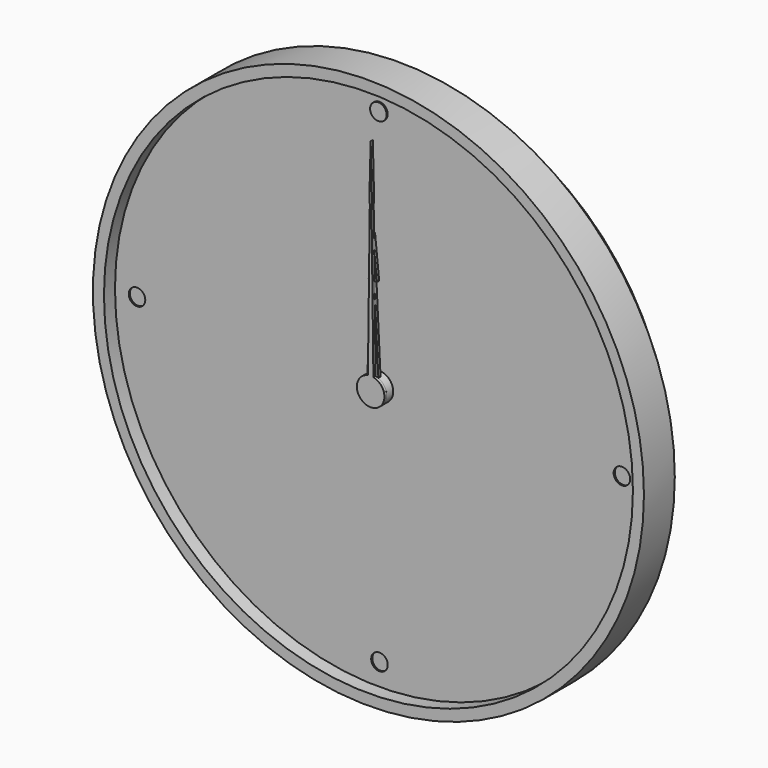
from build123d import *

# Parameters (mm, degrees)
F0_R      = 100
F1_DEPTH  = 24
F2_SIZE   = 10
F3_T      = -4
F4_R      = 5
F4_R_2    = 3
F5_DEPTH  = 2
F6_DEPTH  = 19
F7_DEPTH  = 8
F9_DEPTH  = 4
F11_DEPTH = 4
F12_R     = 5
F12_R_2   = 3
F13_DEPTH = 2
F14_R     = 3
F15_DEPTH = 4
F16_R     = 7.5
F17_DEPTH = 4
F18_R     = 3
F19_DEPTH = 2
F20_R     = 98
F20_R_2   = 5
F21_DEPTH = 1
F23_R     = 5
F23_R_2   = 3
F24_DEPTH = 2
F25_R     = 3
F26_DEPTH = 0.5
F27_DEPTH = 1
F28_R     = 5
F28_R_2   = 3
F29_DEPTH = 5
F30_R     = 3
F31_DEPTH = 1
F33_DEPTH = 1


with BuildPart() as f1:
    # F0 (on Front) → F1 (new body)
    with BuildSketch(Plane.XZ):
        Circle(F0_R)
    extrude(amount=F1_DEPTH)

    # F2
    f2_edges = [f1.edges().sort_by_distance(p)[0] for p in [
        (-100, 0, 0),
    ]]
    chamfer(f2_edges, length=F2_SIZE)

    # F3
    f3_openings = [f1.faces().sort_by_distance(p)[0] for p in [
        (0, -24, 0),
    ]]
    offset(amount=F3_T, openings=f3_openings)

    # F4 (on face) → F5 (join)
    with BuildSketch(Plane.XZ.offset(4)):
        Circle(F4_R)
        Circle(F4_R_2, mode=Mode.SUBTRACT)
        with Locations((40, 0)):
            Circle(F4_R)
        with Locations((40, 0)):
            Circle(F4_R_2, mode=Mode.SUBTRACT)
    extrude(amount=F5_DEPTH)


with BuildPart() as f6:
    # F6 (new): a face of the model
    f6_faces = [f1.part.faces().sort_by_distance(p)[0] for p in [
        (0, -4, 0),
    ]]
    extrude(f6_faces, amount=F6_DEPTH)

    # F8 (on face) → F9 (join)
    with BuildSketch(Plane.XZ.offset(6)):
        with BuildLine():
            ThreePointArc((9.2729637667, -1.3794085621), (9.3494561423, -0.6915886375), (9.375, 0))
            ThreePointArc((9.375, 0), (9.3494561423, 0.6915886375), (9.2729637667, 1.3794085621))
            ThreePointArc((9.2729637667, 1.3794085621), (8.9161548403, 2.8970343223), (8.3127812852, 4.3345463782))
            ThreePointArc((8.3127812852, 4.3345463782), (7.5845343223, 5.5104867402), (6.6911892658, 6.566476316))
            ThreePointArc((6.6911892658, 6.566476316), (5.5104867402, 7.5845343223), (4.1773988938, 8.3928519278))
            ThreePointArc((4.1773988938, 8.3928519278), (2.8970343223, 8.9161548403), (1.5536078905, 9.2453733036))
            ThreePointArc((1.5536078905, 9.2453733036), (0, 9.375), (-1.5536078905, 9.2453733036))
            ThreePointArc((-1.5536078905, 9.2453733036), (-2.8970343223, 8.9161548403), (-4.1773988938, 8.3928519278))
            ThreePointArc((-4.1773988938, 8.3928519278), (-5.5104867402, 7.5845343223), (-6.6911892658, 6.566476316))
            ThreePointArc((-6.6911892658, 6.566476316), (-7.5845343223, 5.5104867402), (-8.3127812852, 4.3345463782))
            ThreePointArc((-8.3127812852, 4.3345463782), (-8.9161548403, 2.8970343223), (-9.2729637667, 1.3794085621))
            ThreePointArc((-9.2729637667, 1.3794085621), (-9.375, 0), (-9.2729637667, -1.3794085621))
            ThreePointArc((-9.2729637667, -1.3794085621), (-8.9161548403, -2.8970343223), (-8.3127812852, -4.3345463782))
            ThreePointArc((-8.3127812852, -4.3345463782), (-7.5845343223, -5.5104867402), (-6.6911892658, -6.566476316))
            ThreePointArc((-6.6911892658, -6.566476316), (-5.5104867402, -7.5845343223), (-4.1773988938, -8.3928519278))
            ThreePointArc((-4.1773988938, -8.3928519278), (-2.8970343223, -8.9161548403), (-1.5536078905, -9.2453733036))
            ThreePointArc((-1.5536078905, -9.2453733036), (0, -9.375), (1.5536078905, -9.2453733036))
            ThreePointArc((1.5536078905, -9.2453733036), (2.8970343223, -8.9161548403), (4.1773988938, -8.3928519278))
            ThreePointArc((4.1773988938, -8.3928519278), (5.5104867402, -7.5845343223), (6.6911892658, -6.566476316))
            ThreePointArc((6.6911892658, -6.566476316), (7.5845343223, -5.5104867402), (8.3127812852, -4.3345463782))
            ThreePointArc((8.3127812852, -4.3345463782), (8.9161548403, -2.8970343223), (9.2729637667, -1.3794085621))
        make_face()
        with BuildLine():
            ThreePointArc((8.3127812852, 4.3345463782), (8.9161548403, 2.8970343223), (9.2729637667, 1.3794085621))
            Line((9.2729637667, 1.3794085621), (11.1823199426, 2.3946312492))
            Line((11.1823199426, 2.3946312492), (10.8182678729, 3.515068311))
            Line((10.8182678729, 3.515068311), (10.4542158031, 4.6355053728))
            Line((10.4542158031, 4.6355053728), (8.3127812852, 4.3345463782))
        make_face()
        with BuildLine():
            Line((11.1823199426, -2.3946312492), (9.2729637667, -1.3794085621))
            ThreePointArc((9.2729637667, -1.3794085621), (8.9161548403, -2.8970343223), (8.3127812852, -4.3345463782))
            Line((8.3127812852, -4.3345463782), (10.4542158031, -4.6355053728))
            Line((10.4542158031, -4.6355053728), (10.8182678729, -3.515068311))
            Line((10.8182678729, -3.515068311), (11.1823199426, -2.3946312492))
        make_face()
        with BuildLine():
            ThreePointArc((4.1773988938, 8.3928519278), (5.5104867402, 7.5845343223), (6.6911892658, 6.566476316))
            Line((6.6911892658, 6.566476316), (7.6391579371, 8.5101001246))
            Line((7.6391579371, 8.5101001246), (6.6860572448, 9.202568311))
            Line((6.6860572448, 9.202568311), (5.7329565525, 9.8950364974))
            Line((5.7329565525, 9.8950364974), (4.1773988938, 8.3928519278))
        make_face()
        with BuildLine():
            Line((7.6391579371, -8.5101001246), (6.6911892658, -6.566476316))
            ThreePointArc((6.6911892658, -6.566476316), (5.5104867402, -7.5845343223), (4.1773988938, -8.3928519278))
            Line((4.1773988938, -8.3928519278), (5.7329565525, -9.8950364974))
            Line((5.7329565525, -9.8950364974), (6.6860572448, -9.202568311))
            Line((6.6860572448, -9.202568311), (7.6391579371, -8.5101001246))
        make_face()
        with BuildLine():
            ThreePointArc((-1.5536078905, 9.2453733036), (0, 9.375), (1.5536078905, 9.2453733036))
            Line((1.5536078905, 9.2453733036), (1.1780972451, 11.375))
            Line((1.1780972451, 11.375), (0, 11.375))
            Line((0, 11.375), (-1.1780972451, 11.375))
            Line((-1.1780972451, 11.375), (-1.5536078905, 9.2453733036))
        make_face()
        with BuildLine():
            Line((1.1780972451, -11.375), (1.5536078905, -9.2453733036))
            ThreePointArc((1.5536078905, -9.2453733036), (0, -9.375), (-1.5536078905, -9.2453733036))
            Line((-1.5536078905, -9.2453733036), (-1.1780972451, -11.375))
            Line((-1.1780972451, -11.375), (0, -11.375))
            Line((0, -11.375), (1.1780972451, -11.375))
        make_face()
        with BuildLine():
            ThreePointArc((-6.6911892658, 6.566476316), (-5.5104867402, 7.5845343223), (-4.1773988938, 8.3928519278))
            Line((-4.1773988938, 8.3928519278), (-5.7329565525, 9.8950364974))
            Line((-5.7329565525, 9.8950364974), (-6.6860572448, 9.202568311))
            Line((-6.6860572448, 9.202568311), (-7.6391579371, 8.5101001246))
            Line((-7.6391579371, 8.5101001246), (-6.6911892658, 6.566476316))
        make_face()
        with BuildLine():
            Line((-5.7329565525, -9.8950364974), (-4.1773988938, -8.3928519278))
            ThreePointArc((-4.1773988938, -8.3928519278), (-5.5104867402, -7.5845343223), (-6.6911892658, -6.566476316))
            Line((-6.6911892658, -6.566476316), (-7.6391579371, -8.5101001246))
            Line((-7.6391579371, -8.5101001246), (-6.6860572448, -9.202568311))
            Line((-6.6860572448, -9.202568311), (-5.7329565525, -9.8950364974))
        make_face()
        with BuildLine():
            ThreePointArc((-9.2729637667, 1.3794085621), (-8.9161548403, 2.8970343223), (-8.3127812852, 4.3345463782))
            Line((-8.3127812852, 4.3345463782), (-10.4542158031, 4.6355053728))
            Line((-10.4542158031, 4.6355053728), (-10.8182678729, 3.515068311))
            Line((-10.8182678729, 3.515068311), (-11.1823199426, 2.3946312492))
            Line((-11.1823199426, 2.3946312492), (-9.2729637667, 1.3794085621))
        make_face()
        with BuildLine():
            Line((-10.4542158031, -4.6355053728), (-8.3127812852, -4.3345463782))
            ThreePointArc((-8.3127812852, -4.3345463782), (-8.9161548403, -2.8970343223), (-9.2729637667, -1.3794085621))
            Line((-9.2729637667, -1.3794085621), (-11.1823199426, -2.3946312492))
            Line((-11.1823199426, -2.3946312492), (-10.8182678729, -3.515068311))
            Line((-10.8182678729, -3.515068311), (-10.4542158031, -4.6355053728))
        make_face()
    extrude(amount=F9_DEPTH)

    # F32 (on face) → F33 (join)
    with BuildSketch(Plane.XZ.offset(23)):
        with BuildLine():
            ThreePointArc((-1, 4.8989794856), (-3.1622776602, -3.8729833462), (5, 0))
            ThreePointArc((5, 0), (3.8729833462, 3.1622776602), (1, 4.8989794856))
            ThreePointArc((1, 4.8989794856), (0, 5), (-1, 4.8989794856))
        make_face()
        with BuildLine():
            ThreePointArc((-1, 4.8989794856), (0, 5), (1, 4.8989794856))
            Line((1, 4.8989794856), (0.3, 60.0062509769))
            Line((0.3, 60.0062509769), (0.5, 60.0062509769))
            Line((0.5, 60.0062509769), (0, 80))
            Line((0, 80), (-0.5, 60.0062509769))
            Line((-0.5, 60.0062509769), (-0.3, 60.0062509769))
            Line((-0.3, 60.0062509769), (-1, 4.8989794856))
        make_face()
    extrude(amount=-F33_DEPTH)


with BuildPart() as f7:
    # F7 (new): a face of the model
    f7_faces = [f1.part.faces().sort_by_distance(p)[0] for p in [
        (40, -4, 0),
    ]]
    extrude(f7_faces, amount=F7_DEPTH)

    # F10 (on face) → F11 (join)
    with BuildSketch(Plane.XZ.offset(6)):
        with BuildLine():
            ThreePointArc((68.0829066802, -1.5381733945), (68.1144747006, -0.7693746225), (68.125, 0))
            ThreePointArc((68.125, 0), (68.1144747006, 0.7693746225), (68.0829066802, 1.5381733945))
            ThreePointArc((68.0829066802, 1.5381733945), (67.9709283072, 2.9398630294), (67.7890320221, 4.3342039956))
            ThreePointArc((67.7890320221, 4.3342039956), (67.5104012706, 5.8475163042), (67.1494235596, 7.3433252263))
            ThreePointArc((67.1494235596, 7.3433252263), (66.7484645208, 8.6911029668), (66.280643318, 10.0171558733))
            ThreePointArc((66.280643318, 10.0171558733), (65.6934659962, 11.4394680865), (65.0293803521, 12.8275385085))
            ThreePointArc((65.0293803521, 12.8275385085), (64.3569644814, 14.0625), (63.6236643925, 15.2623099717))
            ThreePointArc((63.6236643925, 15.2623099717), (62.7536029668, 16.5314602207), (61.815433119, 17.7511268046))
            ThreePointArc((61.815433119, 17.7511268046), (60.9009482166, 18.8192983038), (59.934217974, 19.8404278876))
            ThreePointArc((59.934217974, 19.8404278876), (58.8192983038, 20.9009482166), (57.6480467764, 21.8989056799))
            ThreePointArc((57.6480467764, 21.8989056799), (56.5314602207, 22.7536029668), (55.3735505752, 23.5514238999))
            ThreePointArc((55.3735505752, 23.5514238999), (54.0625, 24.3569644814), (52.709356105, 25.0895972944))
            ThreePointArc((52.709356105, 25.0895972944), (51.4394680865, 25.6934659962), (50.1409852457, 26.2331096755))
            ThreePointArc((50.1409852457, 26.2331096755), (48.6911029668, 26.7484645208), (47.2152055856, 27.1837531139))
            ThreePointArc((47.2152055856, 27.1837531139), (45.8475163042, 27.5104012706), (44.4652101991, 27.7682826779))
            ThreePointArc((44.4652101991, 27.7682826779), (42.9398630294, 27.9709283072), (41.4057159597, 28.0898484802))
            ThreePointArc((41.4057159597, 28.0898484802), (40, 28.125), (38.5942840403, 28.0898484802))
            ThreePointArc((38.5942840403, 28.0898484802), (37.0601369706, 27.9709283072), (35.5347898009, 27.7682826779))
            ThreePointArc((35.5347898009, 27.7682826779), (34.1524836958, 27.5104012706), (32.7847944144, 27.1837531139))
            ThreePointArc((32.7847944144, 27.1837531139), (31.3088970332, 26.7484645208), (29.8590147543, 26.2331096755))
            ThreePointArc((29.8590147543, 26.2331096755), (28.5605319135, 25.6934659962), (27.290643895, 25.0895972944))
            ThreePointArc((27.290643895, 25.0895972944), (25.9375, 24.3569644814), (24.6264494248, 23.5514238999))
            ThreePointArc((24.6264494248, 23.5514238999), (23.4685397793, 22.7536029668), (22.3519532236, 21.8989056799))
            ThreePointArc((22.3519532236, 21.8989056799), (21.1807016962, 20.9009482166), (20.065782026, 19.8404278876))
            ThreePointArc((20.065782026, 19.8404278876), (19.0990517834, 18.8192983038), (18.184566881, 17.7511268046))
            ThreePointArc((18.184566881, 17.7511268046), (17.2463970332, 16.5314602207), (16.3763356075, 15.2623099717))
            ThreePointArc((16.3763356075, 15.2623099717), (15.6430355186, 14.0625), (14.9706196479, 12.8275385085))
            ThreePointArc((14.9706196479, 12.8275385085), (14.3065340038, 11.4394680865), (13.719356682, 10.0171558733))
            ThreePointArc((13.719356682, 10.0171558733), (13.2515354792, 8.6911029668), (12.8505764404, 7.3433252263))
            ThreePointArc((12.8505764404, 7.3433252263), (12.4895987294, 5.8475163042), (12.2109679779, 4.3342039956))
            ThreePointArc((12.2109679779, 4.3342039956), (12.0290716928, 2.9398630294), (11.9170933198, 1.5381733945))
            ThreePointArc((11.9170933198, 1.5381733945), (11.875, 0), (11.9170933198, -1.5381733945))
            ThreePointArc((11.9170933198, -1.5381733945), (12.0290716928, -2.9398630294), (12.2109679779, -4.3342039956))
            ThreePointArc((12.2109679779, -4.3342039956), (12.4895987294, -5.8475163042), (12.8505764404, -7.3433252263))
            ThreePointArc((12.8505764404, -7.3433252263), (13.2515354792, -8.6911029668), (13.719356682, -10.0171558733))
            ThreePointArc((13.719356682, -10.0171558733), (14.3065340038, -11.4394680865), (14.9706196479, -12.8275385085))
            ThreePointArc((14.9706196479, -12.8275385085), (15.6430355186, -14.0625), (16.3763356075, -15.2623099717))
            ThreePointArc((16.3763356075, -15.2623099717), (17.2463970332, -16.5314602207), (18.184566881, -17.7511268046))
            ThreePointArc((18.184566881, -17.7511268046), (19.0990517834, -18.8192983038), (20.065782026, -19.8404278876))
            ThreePointArc((20.065782026, -19.8404278876), (21.1807016962, -20.9009482166), (22.3519532236, -21.8989056799))
            ThreePointArc((22.3519532236, -21.8989056799), (23.4685397793, -22.7536029668), (24.6264494248, -23.5514238999))
            ThreePointArc((24.6264494248, -23.5514238999), (25.9375, -24.3569644814), (27.290643895, -25.0895972944))
            ThreePointArc((27.290643895, -25.0895972944), (28.5605319135, -25.6934659962), (29.8590147543, -26.2331096755))
            ThreePointArc((29.8590147543, -26.2331096755), (31.3088970332, -26.7484645208), (32.7847944144, -27.1837531139))
            ThreePointArc((32.7847944144, -27.1837531139), (34.1524836958, -27.5104012706), (35.5347898009, -27.7682826779))
            ThreePointArc((35.5347898009, -27.7682826779), (37.0601369706, -27.9709283072), (38.5942840403, -28.0898484802))
            ThreePointArc((38.5942840403, -28.0898484802), (40, -28.125), (41.4057159597, -28.0898484802))
            ThreePointArc((41.4057159597, -28.0898484802), (42.9398630294, -27.9709283072), (44.4652101991, -27.7682826779))
            ThreePointArc((44.4652101991, -27.7682826779), (45.8475163042, -27.5104012706), (47.2152055856, -27.1837531139))
            ThreePointArc((47.2152055856, -27.1837531139), (48.6911029668, -26.7484645208), (50.1409852457, -26.2331096755))
            ThreePointArc((50.1409852457, -26.2331096755), (51.4394680865, -25.6934659962), (52.709356105, -25.0895972944))
            ThreePointArc((52.709356105, -25.0895972944), (54.0625, -24.3569644814), (55.3735505752, -23.5514238999))
            ThreePointArc((55.3735505752, -23.5514238999), (56.5314602207, -22.7536029668), (57.6480467764, -21.8989056799))
            ThreePointArc((57.6480467764, -21.8989056799), (58.8192983038, -20.9009482166), (59.934217974, -19.8404278876))
            ThreePointArc((59.934217974, -19.8404278876), (60.9009482166, -18.8192983038), (61.815433119, -17.7511268046))
            ThreePointArc((61.815433119, -17.7511268046), (62.7536029668, -16.5314602207), (63.6236643925, -15.2623099717))
            ThreePointArc((63.6236643925, -15.2623099717), (64.3569644814, -14.0625), (65.0293803521, -12.8275385085))
            ThreePointArc((65.0293803521, -12.8275385085), (65.6934659962, -11.4394680865), (66.280643318, -10.0171558733))
            ThreePointArc((66.280643318, -10.0171558733), (66.7484645208, -8.6911029668), (67.1494235596, -7.3433252263))
            ThreePointArc((67.1494235596, -7.3433252263), (67.5104012706, -5.8475163042), (67.7890320221, -4.3342039956))
            ThreePointArc((67.7890320221, -4.3342039956), (67.9709283072, -2.9398630294), (68.0829066802, -1.5381733945))
        make_face()
        with BuildLine():
            ThreePointArc((68.0829066802, 1.5381733945), (68.1144747006, 0.7693746225), (68.125, 0))
            ThreePointArc((68.125, 0), (68.1144747006, -0.7693746225), (68.0829066802, -1.5381733945))
            Line((68.0829066802, -1.5381733945), (70.125, -1.1780972451))
            Line((70.125, -1.1780972451), (70.125, 0))
            Line((70.125, 0), (70.125, 1.1780972451))
            Line((70.125, 1.1780972451), (68.0829066802, 1.5381733945))
        make_face()
        with BuildLine():
            ThreePointArc((67.1494235596, 7.3433252263), (67.5104012706, 5.8475163042), (67.7890320221, 4.3342039956))
            Line((67.7890320221, 4.3342039956), (69.7116366623, 5.1109866922))
            Line((69.7116366623, 5.1109866922), (69.4666964721, 6.2633396859))
            Line((69.4666964721, 6.2633396859), (69.2217562819, 7.4156926796))
            Line((69.2217562819, 7.4156926796), (67.1494235596, 7.3433252263))
        make_face()
        with BuildLine():
            Line((69.7116366623, -5.1109866922), (67.7890320221, -4.3342039956))
            ThreePointArc((67.7890320221, -4.3342039956), (67.5104012706, -5.8475163042), (67.1494235596, -7.3433252263))
            Line((67.1494235596, -7.3433252263), (69.2217562819, -7.4156926796))
            Line((69.2217562819, -7.4156926796), (69.4666964721, -6.2633396859))
            Line((69.4666964721, -6.2633396859), (69.7116366623, -5.1109866922))
        make_face()
        with BuildLine():
            ThreePointArc((65.0293803521, 12.8275385085), (65.6934659962, 11.4394680865), (66.280643318, 10.0171558733))
            Line((66.280643318, 10.0171558733), (67.9997322302, 11.1766959857))
            Line((67.9997322302, 11.1766959857), (67.5205569115, 12.2529413727))
            Line((67.5205569115, 12.2529413727), (67.0413815928, 13.3291867596))
            Line((67.0413815928, 13.3291867596), (65.0293803521, 12.8275385085))
        make_face()
        with BuildLine():
            Line((67.9997322302, -11.1766959857), (66.280643318, -10.0171558733))
            ThreePointArc((66.280643318, -10.0171558733), (65.6934659962, -11.4394680865), (65.0293803521, -12.8275385085))
            Line((65.0293803521, -12.8275385085), (67.0413815928, -13.3291867596))
            Line((67.0413815928, -13.3291867596), (67.5205569115, -12.2529413727))
            Line((67.5205569115, -12.2529413727), (67.9997322302, -11.1766959857))
        make_face()
        with BuildLine():
            ThreePointArc((61.815433119, 17.7511268046), (62.7536029668, 16.5314602207), (63.6236643925, 15.2623099717))
            Line((63.6236643925, 15.2623099717), (65.064105142, 16.753930033))
            Line((65.064105142, 16.753930033), (64.3716369555, 17.7070307253))
            Line((64.3716369555, 17.7070307253), (63.6791687691, 18.6601314176))
            Line((63.6791687691, 18.6601314176), (61.815433119, 17.7511268046))
        make_face()
        with BuildLine():
            Line((65.064105142, -16.753930033), (63.6236643925, -15.2623099717))
            ThreePointArc((63.6236643925, -15.2623099717), (62.7536029668, -16.5314602207), (61.815433119, -17.7511268046))
            Line((61.815433119, -17.7511268046), (63.6791687691, -18.6601314176))
            Line((63.6791687691, -18.6601314176), (64.3716369555, -17.7070307253))
            Line((64.3716369555, -17.7070307253), (65.064105142, -16.753930033))
        make_face()
        with BuildLine():
            ThreePointArc((57.6480467764, 21.8989056799), (58.8192983038, 20.9009482166), (59.934217974, 19.8404278876))
            Line((59.934217974, 19.8404278876), (61.0330563882, 21.5989369435))
            Line((61.0330563882, 21.5989369435), (60.1575595166, 22.3872378675))
            Line((60.1575595166, 22.3872378675), (59.282062645, 23.1755387915))
            Line((59.282062645, 23.1755387915), (57.6480467764, 21.8989056799))
        make_face()
        with BuildLine():
            Line((61.0330563882, -21.5989369435), (59.934217974, -19.8404278876))
            ThreePointArc((59.934217974, -19.8404278876), (58.8192983038, -20.9009482166), (57.6480467764, -21.8989056799))
            Line((57.6480467764, -21.8989056799), (59.282062645, -23.1755387915))
            Line((59.282062645, -23.1755387915), (60.1575595166, -22.3872378675))
            Line((60.1575595166, -22.3872378675), (61.0330563882, -21.5989369435))
        make_face()
        with BuildLine():
            ThreePointArc((52.709356105, 25.0895972944), (54.0625, 24.3569644814), (55.3735505752, 23.5514238999))
            Line((55.3735505752, 23.5514238999), (56.0827621424, 25.4999666665))
            Line((56.0827621424, 25.4999666665), (55.0625, 26.089015289))
            Line((55.0625, 26.089015289), (54.0422378576, 26.6780639116))
            Line((54.0422378576, 26.6780639116), (52.709356105, 25.0895972944))
        make_face()
        with BuildLine():
            Line((56.0827621424, -25.4999666665), (55.3735505752, -23.5514238999))
            ThreePointArc((55.3735505752, -23.5514238999), (54.0625, -24.3569644814), (52.709356105, -25.0895972944))
            Line((52.709356105, -25.0895972944), (54.0422378576, -26.6780639116))
            Line((54.0422378576, -26.6780639116), (55.0625, -26.089015289))
            Line((55.0625, -26.089015289), (56.0827621424, -25.4999666665))
        make_face()
        with BuildLine():
            ThreePointArc((47.2152055856, 27.1837531139), (48.6911029668, 26.7484645208), (50.1409852457, 26.2331096755))
            Line((50.1409852457, 26.2331096755), (50.4295740173, 28.2865254836))
            Line((50.4295740173, 28.2865254836), (49.3091369555, 28.6505775534))
            Line((49.3091369555, 28.6505775534), (48.1886998938, 29.0146296232))
            Line((48.1886998938, 29.0146296232), (47.2152055856, 27.1837531139))
        make_face()
        with BuildLine():
            Line((50.4295740173, -28.2865254836), (50.1409852457, -26.2331096755))
            ThreePointArc((50.1409852457, -26.2331096755), (48.6911029668, -26.7484645208), (47.2152055856, -27.1837531139))
            Line((47.2152055856, -27.1837531139), (48.1886998938, -29.0146296232))
            Line((48.1886998938, -29.0146296232), (49.3091369555, -28.6505775534))
            Line((49.3091369555, -28.6505775534), (50.4295740173, -28.2865254836))
        make_face()
        with BuildLine():
            ThreePointArc((41.4057159597, 28.0898484802), (42.9398630294, 27.9709283072), (44.4652101991, 27.7682826779))
            Line((44.4652101991, 27.7682826779), (44.3205634611, 29.8368274034))
            Line((44.3205634611, 29.8368274034), (43.1489199559, 29.959972098))
            Line((43.1489199559, 29.959972098), (41.9772764508, 30.0831167926))
            Line((41.9772764508, 30.0831167926), (41.4057159597, 28.0898484802))
        make_face()
        with BuildLine():
            Line((44.3205634611, -29.8368274034), (44.4652101991, -27.7682826779))
            ThreePointArc((44.4652101991, -27.7682826779), (42.9398630294, -27.9709283072), (41.4057159597, -28.0898484802))
            Line((41.4057159597, -28.0898484802), (41.9772764508, -30.0831167926))
            Line((41.9772764508, -30.0831167926), (43.1489199559, -29.959972098))
            Line((43.1489199559, -29.959972098), (44.3205634611, -29.8368274034))
        make_face()
        with BuildLine():
            ThreePointArc((35.5347898009, 27.7682826779), (37.0601369706, 27.9709283072), (38.5942840403, 28.0898484802))
            Line((38.5942840403, 28.0898484802), (38.0227235492, 30.0831167926))
            Line((38.0227235492, 30.0831167926), (36.8510800441, 29.959972098))
            Line((36.8510800441, 29.959972098), (35.6794365389, 29.8368274034))
            Line((35.6794365389, 29.8368274034), (35.5347898009, 27.7682826779))
        make_face()
        with BuildLine():
            Line((38.0227235492, -30.0831167926), (38.5942840403, -28.0898484802))
            ThreePointArc((38.5942840403, -28.0898484802), (37.0601369706, -27.9709283072), (35.5347898009, -27.7682826779))
            Line((35.5347898009, -27.7682826779), (35.6794365389, -29.8368274034))
            Line((35.6794365389, -29.8368274034), (36.8510800441, -29.959972098))
            Line((36.8510800441, -29.959972098), (38.0227235492, -30.0831167926))
        make_face()
        with BuildLine():
            ThreePointArc((29.8590147543, 26.2331096755), (31.3088970332, 26.7484645208), (32.7847944144, 27.1837531139))
            Line((32.7847944144, 27.1837531139), (31.8113001062, 29.0146296232))
            Line((31.8113001062, 29.0146296232), (30.6908630445, 28.6505775534))
            Line((30.6908630445, 28.6505775534), (29.5704259827, 28.2865254836))
            Line((29.5704259827, 28.2865254836), (29.8590147543, 26.2331096755))
        make_face()
        with BuildLine():
            Line((31.8113001062, -29.0146296232), (32.7847944144, -27.1837531139))
            ThreePointArc((32.7847944144, -27.1837531139), (31.3088970332, -26.7484645208), (29.8590147543, -26.2331096755))
            Line((29.8590147543, -26.2331096755), (29.5704259827, -28.2865254836))
            Line((29.5704259827, -28.2865254836), (30.6908630445, -28.6505775534))
            Line((30.6908630445, -28.6505775534), (31.8113001062, -29.0146296232))
        make_face()
        with BuildLine():
            ThreePointArc((24.6264494248, 23.5514238999), (25.9375, 24.3569644814), (27.290643895, 25.0895972944))
            Line((27.290643895, 25.0895972944), (25.9577621424, 26.6780639116))
            Line((25.9577621424, 26.6780639116), (24.9375, 26.089015289))
            Line((24.9375, 26.089015289), (23.9172378576, 25.4999666665))
            Line((23.9172378576, 25.4999666665), (24.6264494248, 23.5514238999))
        make_face()
        with BuildLine():
            Line((25.9577621424, -26.6780639116), (27.290643895, -25.0895972944))
            ThreePointArc((27.290643895, -25.0895972944), (25.9375, -24.3569644814), (24.6264494248, -23.5514238999))
            Line((24.6264494248, -23.5514238999), (23.9172378576, -25.4999666665))
            Line((23.9172378576, -25.4999666665), (24.9375, -26.089015289))
            Line((24.9375, -26.089015289), (25.9577621424, -26.6780639116))
        make_face()
        with BuildLine():
            ThreePointArc((20.065782026, 19.8404278876), (21.1807016962, 20.9009482166), (22.3519532236, 21.8989056799))
            Line((22.3519532236, 21.8989056799), (20.717937355, 23.1755387915))
            Line((20.717937355, 23.1755387915), (19.8424404834, 22.3872378675))
            Line((19.8424404834, 22.3872378675), (18.9669436118, 21.5989369435))
            Line((18.9669436118, 21.5989369435), (20.065782026, 19.8404278876))
        make_face()
        with BuildLine():
            Line((20.717937355, -23.1755387915), (22.3519532236, -21.8989056799))
            ThreePointArc((22.3519532236, -21.8989056799), (21.1807016962, -20.9009482166), (20.065782026, -19.8404278876))
            Line((20.065782026, -19.8404278876), (18.9669436118, -21.5989369435))
            Line((18.9669436118, -21.5989369435), (19.8424404834, -22.3872378675))
            Line((19.8424404834, -22.3872378675), (20.717937355, -23.1755387915))
        make_face()
        with BuildLine():
            ThreePointArc((16.3763356075, 15.2623099717), (17.2463970332, 16.5314602207), (18.184566881, 17.7511268046))
            Line((18.184566881, 17.7511268046), (16.3208312309, 18.6601314176))
            Line((16.3208312309, 18.6601314176), (15.6283630445, 17.7070307253))
            Line((15.6283630445, 17.7070307253), (14.935894858, 16.753930033))
            Line((14.935894858, 16.753930033), (16.3763356075, 15.2623099717))
        make_face()
        with BuildLine():
            Line((16.3208312309, -18.6601314176), (18.184566881, -17.7511268046))
            ThreePointArc((18.184566881, -17.7511268046), (17.2463970332, -16.5314602207), (16.3763356075, -15.2623099717))
            Line((16.3763356075, -15.2623099717), (14.935894858, -16.753930033))
            Line((14.935894858, -16.753930033), (15.6283630445, -17.7070307253))
            Line((15.6283630445, -17.7070307253), (16.3208312309, -18.6601314176))
        make_face()
        with BuildLine():
            ThreePointArc((13.719356682, 10.0171558733), (14.3065340038, 11.4394680865), (14.9706196479, 12.8275385085))
            Line((14.9706196479, 12.8275385085), (12.9586184072, 13.3291867596))
            Line((12.9586184072, 13.3291867596), (12.4794430885, 12.2529413727))
            Line((12.4794430885, 12.2529413727), (12.0002677698, 11.1766959857))
            Line((12.0002677698, 11.1766959857), (13.719356682, 10.0171558733))
        make_face()
        with BuildLine():
            Line((12.9586184072, -13.3291867596), (14.9706196479, -12.8275385085))
            ThreePointArc((14.9706196479, -12.8275385085), (14.3065340038, -11.4394680865), (13.719356682, -10.0171558733))
            Line((13.719356682, -10.0171558733), (12.0002677698, -11.1766959857))
            Line((12.0002677698, -11.1766959857), (12.4794430885, -12.2529413727))
            Line((12.4794430885, -12.2529413727), (12.9586184072, -13.3291867596))
        make_face()
        with BuildLine():
            ThreePointArc((12.2109679779, 4.3342039956), (12.4895987294, 5.8475163042), (12.8505764404, 7.3433252263))
            Line((12.8505764404, 7.3433252263), (10.7782437181, 7.4156926796))
            Line((10.7782437181, 7.4156926796), (10.5333035279, 6.2633396859))
            Line((10.5333035279, 6.2633396859), (10.2883633377, 5.1109866922))
            Line((10.2883633377, 5.1109866922), (12.2109679779, 4.3342039956))
        make_face()
        with BuildLine():
            Line((10.7782437181, -7.4156926796), (12.8505764404, -7.3433252263))
            ThreePointArc((12.8505764404, -7.3433252263), (12.4895987294, -5.8475163042), (12.2109679779, -4.3342039956))
            Line((12.2109679779, -4.3342039956), (10.2883633377, -5.1109866922))
            Line((10.2883633377, -5.1109866922), (10.5333035279, -6.2633396859))
            Line((10.5333035279, -6.2633396859), (10.7782437181, -7.4156926796))
        make_face()
        with BuildLine():
            ThreePointArc((11.9170933198, -1.5381733945), (11.875, 0), (11.9170933198, 1.5381733945))
            Line((11.9170933198, 1.5381733945), (9.875, 1.1780972451))
            Line((9.875, 1.1780972451), (9.875, 0))
            Line((9.875, 0), (9.875, -1.1780972451))
            Line((9.875, -1.1780972451), (11.9170933198, -1.5381733945))
        make_face()
    extrude(amount=F11_DEPTH)

    # F16 (on face) → F17 (join)
    with BuildSketch(Plane.XZ.offset(12)):
        with Locations((40, 0)):
            Circle(F16_R)
    extrude(amount=F17_DEPTH)

    # F18 (on face) → F19 (join)
    with BuildSketch(Plane.XZ.offset(16)):
        with Locations((40, 0)):
            Circle(F18_R)
    extrude(amount=F19_DEPTH)


with BuildPart() as f13:
    # F12 (on face) → F13 (new body)
    with BuildSketch(Plane.XZ.offset(10)):
        Circle(F12_R)
        Circle(F12_R_2, mode=Mode.SUBTRACT)
    extrude(amount=F13_DEPTH)

    # F14 (on face) → F15 (join)
    with BuildSketch(Plane.XZ.offset(12)):
        with BuildLine():
            ThreePointArc((29.9718156995, -1.3001014101), (29.9929530972, -0.6502034357), (30, 0))
            ThreePointArc((30, 0), (29.9929530972, 0.6502034357), (29.9718156995, 1.3001014101))
            ThreePointArc((29.9718156995, 1.3001014101), (29.907520012, 2.3537728718), (29.8061935814, 3.4045299509))
            ThreePointArc((29.8061935814, 3.4045299509), (29.6306502179, 4.6930339512), (29.3994322443, 5.9727199596))
            ThreePointArc((29.3994322443, 5.9727199596), (29.1710976119, 7.0033609157), (28.9066440563, 8.0253304855))
            ThreePointArc((28.9066440563, 8.0253304855), (28.5316954889, 9.2705098312), (28.1031371961, 10.4982703213))
            ThreePointArc((28.1031371961, 10.4982703213), (27.7163859753, 11.480502971), (27.2953170189, 12.448520749))
            ThreePointArc((27.2953170189, 12.448520749), (26.7301957257, 13.6197149922), (26.1148496411, 14.765318426))
            ThreePointArc((26.1148496411, 14.765318426), (25.5792049306, 15.6749569415), (25.0118886885, 16.5651871174))
            ThreePointArc((25.0118886885, 16.5651871174), (24.2705098312, 17.6335575688), (23.4835278178, 18.6687953878))
            ThreePointArc((23.4835278178, 18.6687953878), (22.812178968, 19.4834414499), (22.1125846489, 20.2739636023))
            ThreePointArc((22.1125846489, 20.2739636023), (21.2132034356, 21.2132034356), (20.2739636023, 22.1125846489))
            ThreePointArc((20.2739636023, 22.1125846489), (19.4834414499, 22.812178968), (18.6687953878, 23.4835278178))
            ThreePointArc((18.6687953878, 23.4835278178), (17.6335575688, 24.2705098312), (16.5651871174, 25.0118886885))
            ThreePointArc((16.5651871174, 25.0118886885), (15.6749569415, 25.5792049306), (14.765318426, 26.1148496411))
            ThreePointArc((14.765318426, 26.1148496411), (13.6197149922, 26.7301957257), (12.448520749, 27.2953170189))
            ThreePointArc((12.448520749, 27.2953170189), (11.480502971, 27.7163859753), (10.4982703213, 28.1031371961))
            ThreePointArc((10.4982703213, 28.1031371961), (9.2705098312, 28.5316954889), (8.0253304855, 28.9066440563))
            ThreePointArc((8.0253304855, 28.9066440563), (7.0033609157, 29.1710976119), (5.9727199596, 29.3994322443))
            ThreePointArc((5.9727199596, 29.3994322443), (4.6930339512, 29.6306502179), (3.4045299509, 29.8061935814))
            ThreePointArc((3.4045299509, 29.8061935814), (2.3537728718, 29.907520012), (1.3001014101, 29.9718156995))
            ThreePointArc((1.3001014101, 29.9718156995), (0, 30), (-1.3001014101, 29.9718156995))
            ThreePointArc((-1.3001014101, 29.9718156995), (-2.3537728718, 29.907520012), (-3.4045299509, 29.8061935814))
            ThreePointArc((-3.4045299509, 29.8061935814), (-4.6930339512, 29.6306502179), (-5.9727199596, 29.3994322443))
            ThreePointArc((-5.9727199596, 29.3994322443), (-7.0033609157, 29.1710976119), (-8.0253304855, 28.9066440563))
            ThreePointArc((-8.0253304855, 28.9066440563), (-9.2705098312, 28.5316954889), (-10.4982703213, 28.1031371961))
            ThreePointArc((-10.4982703213, 28.1031371961), (-11.480502971, 27.7163859753), (-12.448520749, 27.2953170189))
            ThreePointArc((-12.448520749, 27.2953170189), (-13.6197149922, 26.7301957257), (-14.765318426, 26.1148496411))
            ThreePointArc((-14.765318426, 26.1148496411), (-15.6749569415, 25.5792049306), (-16.5651871174, 25.0118886885))
            ThreePointArc((-16.5651871174, 25.0118886885), (-17.6335575688, 24.2705098312), (-18.6687953878, 23.4835278178))
            ThreePointArc((-18.6687953878, 23.4835278178), (-19.4834414499, 22.812178968), (-20.2739636023, 22.1125846489))
            ThreePointArc((-20.2739636023, 22.1125846489), (-21.2132034356, 21.2132034356), (-22.1125846489, 20.2739636023))
            ThreePointArc((-22.1125846489, 20.2739636023), (-22.812178968, 19.4834414499), (-23.4835278178, 18.6687953878))
            ThreePointArc((-23.4835278178, 18.6687953878), (-24.2705098312, 17.6335575688), (-25.0118886885, 16.5651871174))
            ThreePointArc((-25.0118886885, 16.5651871174), (-25.5792049306, 15.6749569415), (-26.1148496411, 14.765318426))
            ThreePointArc((-26.1148496411, 14.765318426), (-26.7301957257, 13.6197149922), (-27.2953170189, 12.448520749))
            ThreePointArc((-27.2953170189, 12.448520749), (-27.7163859753, 11.480502971), (-28.1031371961, 10.4982703213))
            ThreePointArc((-28.1031371961, 10.4982703213), (-28.5316954889, 9.2705098312), (-28.9066440563, 8.0253304855))
            ThreePointArc((-28.9066440563, 8.0253304855), (-29.1710976119, 7.0033609157), (-29.3994322443, 5.9727199596))
            ThreePointArc((-29.3994322443, 5.9727199596), (-29.6306502179, 4.6930339512), (-29.8061935814, 3.4045299509))
            ThreePointArc((-29.8061935814, 3.4045299509), (-29.907520012, 2.3537728718), (-29.9718156995, 1.3001014101))
            ThreePointArc((-29.9718156995, 1.3001014101), (-30, 0), (-29.9718156995, -1.3001014101))
            ThreePointArc((-29.9718156995, -1.3001014101), (-29.907520012, -2.3537728718), (-29.8061935814, -3.4045299509))
            ThreePointArc((-29.8061935814, -3.4045299509), (-29.6306502179, -4.6930339512), (-29.3994322443, -5.9727199596))
            ThreePointArc((-29.3994322443, -5.9727199596), (-29.1710976119, -7.0033609157), (-28.9066440563, -8.0253304855))
            ThreePointArc((-28.9066440563, -8.0253304855), (-28.5316954889, -9.2705098312), (-28.1031371961, -10.4982703213))
            ThreePointArc((-28.1031371961, -10.4982703213), (-27.7163859753, -11.480502971), (-27.2953170189, -12.448520749))
            ThreePointArc((-27.2953170189, -12.448520749), (-26.7301957257, -13.6197149922), (-26.1148496411, -14.765318426))
            ThreePointArc((-26.1148496411, -14.765318426), (-25.5792049306, -15.6749569415), (-25.0118886885, -16.5651871174))
            ThreePointArc((-25.0118886885, -16.5651871174), (-24.2705098312, -17.6335575688), (-23.4835278178, -18.6687953878))
            ThreePointArc((-23.4835278178, -18.6687953878), (-22.812178968, -19.4834414499), (-22.1125846489, -20.2739636023))
            ThreePointArc((-22.1125846489, -20.2739636023), (-21.2132034356, -21.2132034356), (-20.2739636023, -22.1125846489))
            ThreePointArc((-20.2739636023, -22.1125846489), (-19.4834414499, -22.812178968), (-18.6687953878, -23.4835278178))
            ThreePointArc((-18.6687953878, -23.4835278178), (-17.6335575688, -24.2705098312), (-16.5651871174, -25.0118886885))
            ThreePointArc((-16.5651871174, -25.0118886885), (-15.6749569415, -25.5792049306), (-14.765318426, -26.1148496411))
            ThreePointArc((-14.765318426, -26.1148496411), (-13.6197149922, -26.7301957257), (-12.448520749, -27.2953170189))
            ThreePointArc((-12.448520749, -27.2953170189), (-11.480502971, -27.7163859753), (-10.4982703213, -28.1031371961))
            ThreePointArc((-10.4982703213, -28.1031371961), (-9.2705098312, -28.5316954889), (-8.0253304855, -28.9066440563))
            ThreePointArc((-8.0253304855, -28.9066440563), (-7.0033609157, -29.1710976119), (-5.9727199596, -29.3994322443))
            ThreePointArc((-5.9727199596, -29.3994322443), (-4.6930339512, -29.6306502179), (-3.4045299509, -29.8061935814))
            ThreePointArc((-3.4045299509, -29.8061935814), (-2.3537728718, -29.907520012), (-1.3001014101, -29.9718156995))
            ThreePointArc((-1.3001014101, -29.9718156995), (0, -30), (1.3001014101, -29.9718156995))
            ThreePointArc((1.3001014101, -29.9718156995), (2.3537728718, -29.907520012), (3.4045299509, -29.8061935814))
            ThreePointArc((3.4045299509, -29.8061935814), (4.6930339512, -29.6306502179), (5.9727199596, -29.3994322443))
            ThreePointArc((5.9727199596, -29.3994322443), (7.0033609157, -29.1710976119), (8.0253304855, -28.9066440563))
            ThreePointArc((8.0253304855, -28.9066440563), (9.2705098312, -28.5316954889), (10.4982703213, -28.1031371961))
            ThreePointArc((10.4982703213, -28.1031371961), (11.480502971, -27.7163859753), (12.448520749, -27.2953170189))
            ThreePointArc((12.448520749, -27.2953170189), (13.6197149922, -26.7301957257), (14.765318426, -26.1148496411))
            ThreePointArc((14.765318426, -26.1148496411), (15.6749569415, -25.5792049306), (16.5651871174, -25.0118886885))
            ThreePointArc((16.5651871174, -25.0118886885), (17.6335575688, -24.2705098312), (18.6687953878, -23.4835278178))
            ThreePointArc((18.6687953878, -23.4835278178), (19.4834414499, -22.812178968), (20.2739636023, -22.1125846489))
            ThreePointArc((20.2739636023, -22.1125846489), (21.2132034356, -21.2132034356), (22.1125846489, -20.2739636023))
            ThreePointArc((22.1125846489, -20.2739636023), (22.812178968, -19.4834414499), (23.4835278178, -18.6687953878))
            ThreePointArc((23.4835278178, -18.6687953878), (24.2705098312, -17.6335575688), (25.0118886885, -16.5651871174))
            ThreePointArc((25.0118886885, -16.5651871174), (25.5792049306, -15.6749569415), (26.1148496411, -14.765318426))
            ThreePointArc((26.1148496411, -14.765318426), (26.7301957257, -13.6197149922), (27.2953170189, -12.448520749))
            ThreePointArc((27.2953170189, -12.448520749), (27.7163859753, -11.480502971), (28.1031371961, -10.4982703213))
            ThreePointArc((28.1031371961, -10.4982703213), (28.5316954889, -9.2705098312), (28.9066440563, -8.0253304855))
            ThreePointArc((28.9066440563, -8.0253304855), (29.1710976119, -7.0033609157), (29.3994322443, -5.9727199596))
            ThreePointArc((29.3994322443, -5.9727199596), (29.6306502179, -4.6930339512), (29.8061935814, -3.4045299509))
            ThreePointArc((29.8061935814, -3.4045299509), (29.907520012, -2.3537728718), (29.9718156995, -1.3001014101))
        make_face()
        Circle(F14_R, mode=Mode.SUBTRACT)
        with BuildLine():
            ThreePointArc((29.9718156995, 1.3001014101), (29.9929530972, 0.6502034357), (30, 0))
            ThreePointArc((30, 0), (29.9929530972, -0.6502034357), (29.9718156995, -1.3001014101))
            Line((29.9718156995, -1.3001014101), (32, -0.9424777961))
            Line((32, -0.9424777961), (32, 0))
            Line((32, 0), (32, 0.9424777961))
            Line((32, 0.9424777961), (29.9718156995, 1.3001014101))
        make_face()
        with BuildLine():
            ThreePointArc((29.3994322443, 5.9727199596), (29.6306502179, 4.6930339512), (29.8061935814, 3.4045299509))
            Line((29.8061935814, 3.4045299509), (31.7534629089, 4.0750285508))
            Line((31.7534629089, 4.0750285508), (31.606026899, 5.0059028813))
            Line((31.606026899, 5.0059028813), (31.4585908892, 5.9367772117))
            Line((31.4585908892, 5.9367772117), (29.3994322443, 5.9727199596))
        make_face()
        with BuildLine():
            Line((31.7534629089, -4.0750285508), (29.8061935814, -3.4045299509))
            ThreePointArc((29.8061935814, -3.4045299509), (29.6306502179, -4.6930339512), (29.3994322443, -5.9727199596))
            Line((29.3994322443, -5.9727199596), (31.4585908892, -5.9367772117))
            Line((31.4585908892, -5.9367772117), (31.606026899, -5.0059028813))
            Line((31.606026899, -5.0059028813), (31.7534629089, -4.0750285508))
        make_face()
        with BuildLine():
            ThreePointArc((28.1031371961, 10.4982703213), (28.5316954889, 9.2705098312), (28.9066440563, 8.0253304855))
            Line((28.9066440563, 8.0253304855), (30.7250501773, 8.9921941706))
            Line((30.7250501773, 8.9921941706), (30.4338085214, 9.88854382))
            Line((30.4338085214, 9.88854382), (30.1425668656, 10.7848934694))
            Line((30.1425668656, 10.7848934694), (28.1031371961, 10.4982703213))
        make_face()
        with BuildLine():
            Line((30.7250501773, -8.9921941706), (28.9066440563, -8.0253304855))
            ThreePointArc((28.9066440563, -8.0253304855), (28.5316954889, -9.2705098312), (28.1031371961, -10.4982703213))
            Line((28.1031371961, -10.4982703213), (30.1425668656, -10.7848934694))
            Line((30.1425668656, -10.7848934694), (30.4338085214, -9.88854382))
            Line((30.4338085214, -9.88854382), (30.7250501773, -8.9921941706))
        make_face()
        with BuildLine():
            ThreePointArc((26.1148496411, 14.765318426), (26.7301957257, 13.6197149922), (27.2953170189, 12.448520749))
            Line((27.2953170189, 12.448520749), (28.9400847397, 13.6879421265))
            Line((28.9400847397, 13.6879421265), (28.512208774, 14.5276959917))
            Line((28.512208774, 14.5276959917), (28.0843328084, 15.3674498569))
            Line((28.0843328084, 15.3674498569), (26.1148496411, 14.765318426))
        make_face()
        with BuildLine():
            Line((28.9400847397, -13.6879421265), (27.2953170189, -12.448520749))
            ThreePointArc((27.2953170189, -12.448520749), (26.7301957257, -13.6197149922), (26.1148496411, -14.765318426))
            Line((26.1148496411, -14.765318426), (28.0843328084, -15.3674498569))
            Line((28.0843328084, -15.3674498569), (28.512208774, -14.5276959917))
            Line((28.512208774, -14.5276959917), (28.9400847397, -13.6879421265))
        make_face()
        with BuildLine():
            ThreePointArc((23.4835278178, 18.6687953878), (24.2705098312, 17.6335575688), (25.0118886885, 16.5651871174))
            Line((25.0118886885, 16.5651871174), (26.4425183691, 18.0466475195))
            Line((26.4425183691, 18.0466475195), (25.88854382, 18.8091280734))
            Line((25.88854382, 18.8091280734), (25.3345692709, 19.5716086272))
            Line((25.3345692709, 19.5716086272), (23.4835278178, 18.6687953878))
        make_face()
        with BuildLine():
            Line((26.4425183691, -18.0466475195), (25.0118886885, -16.5651871174))
            ThreePointArc((25.0118886885, -16.5651871174), (24.2705098312, -17.6335575688), (23.4835278178, -18.6687953878))
            Line((23.4835278178, -18.6687953878), (25.3345692709, -19.5716086272))
            Line((25.3345692709, -19.5716086272), (25.88854382, -18.8091280734))
            Line((25.88854382, -18.8091280734), (26.4425183691, -18.0466475195))
        make_face()
        with BuildLine():
            ThreePointArc((20.2739636023, 22.1125846489), (21.2132034356, 21.2132034356), (22.1125846489, 20.2739636023))
            Line((22.1125846489, 20.2739636023), (23.2938494387, 21.9609845572))
            Line((23.2938494387, 21.9609845572), (22.627416998, 22.627416998))
            Line((22.627416998, 22.627416998), (21.9609845572, 23.2938494387))
            Line((21.9609845572, 23.2938494387), (20.2739636023, 22.1125846489))
        make_face()
        with BuildLine():
            Line((23.2938494387, -21.9609845572), (22.1125846489, -20.2739636023))
            ThreePointArc((22.1125846489, -20.2739636023), (21.2132034356, -21.2132034356), (20.2739636023, -22.1125846489))
            Line((20.2739636023, -22.1125846489), (21.9609845572, -23.2938494387))
            Line((21.9609845572, -23.2938494387), (22.627416998, -22.627416998))
            Line((22.627416998, -22.627416998), (23.2938494387, -21.9609845572))
        make_face()
        with BuildLine():
            ThreePointArc((16.5651871174, 25.0118886885), (17.6335575688, 24.2705098312), (18.6687953878, 23.4835278178))
            Line((18.6687953878, 23.4835278178), (19.5716086272, 25.3345692709))
            Line((19.5716086272, 25.3345692709), (18.8091280734, 25.88854382))
            Line((18.8091280734, 25.88854382), (18.0466475195, 26.4425183691))
            Line((18.0466475195, 26.4425183691), (16.5651871174, 25.0118886885))
        make_face()
        with BuildLine():
            Line((19.5716086272, -25.3345692709), (18.6687953878, -23.4835278178))
            ThreePointArc((18.6687953878, -23.4835278178), (17.6335575688, -24.2705098312), (16.5651871174, -25.0118886885))
            Line((16.5651871174, -25.0118886885), (18.0466475195, -26.4425183691))
            Line((18.0466475195, -26.4425183691), (18.8091280734, -25.88854382))
            Line((18.8091280734, -25.88854382), (19.5716086272, -25.3345692709))
        make_face()
        with BuildLine():
            ThreePointArc((12.448520749, 27.2953170189), (13.6197149922, 26.7301957257), (14.765318426, 26.1148496411))
            Line((14.765318426, 26.1148496411), (15.3674498569, 28.0843328084))
            Line((15.3674498569, 28.0843328084), (14.5276959917, 28.512208774))
            Line((14.5276959917, 28.512208774), (13.6879421265, 28.9400847397))
            Line((13.6879421265, 28.9400847397), (12.448520749, 27.2953170189))
        make_face()
        with BuildLine():
            Line((15.3674498569, -28.0843328084), (14.765318426, -26.1148496411))
            ThreePointArc((14.765318426, -26.1148496411), (13.6197149922, -26.7301957257), (12.448520749, -27.2953170189))
            Line((12.448520749, -27.2953170189), (13.6879421265, -28.9400847397))
            Line((13.6879421265, -28.9400847397), (14.5276959917, -28.512208774))
            Line((14.5276959917, -28.512208774), (15.3674498569, -28.0843328084))
        make_face()
        with BuildLine():
            ThreePointArc((8.0253304855, 28.9066440563), (9.2705098312, 28.5316954889), (10.4982703213, 28.1031371961))
            Line((10.4982703213, 28.1031371961), (10.7848934694, 30.1425668656))
            Line((10.7848934694, 30.1425668656), (9.88854382, 30.4338085214))
            Line((9.88854382, 30.4338085214), (8.9921941706, 30.7250501773))
            Line((8.9921941706, 30.7250501773), (8.0253304855, 28.9066440563))
        make_face()
        with BuildLine():
            Line((10.7848934694, -30.1425668656), (10.4982703213, -28.1031371961))
            ThreePointArc((10.4982703213, -28.1031371961), (9.2705098312, -28.5316954889), (8.0253304855, -28.9066440563))
            Line((8.0253304855, -28.9066440563), (8.9921941706, -30.7250501773))
            Line((8.9921941706, -30.7250501773), (9.88854382, -30.4338085214))
            Line((9.88854382, -30.4338085214), (10.7848934694, -30.1425668656))
        make_face()
        with BuildLine():
            ThreePointArc((3.4045299509, 29.8061935814), (4.6930339512, 29.6306502179), (5.9727199596, 29.3994322443))
            Line((5.9727199596, 29.3994322443), (5.9367772117, 31.4585908892))
            Line((5.9367772117, 31.4585908892), (5.0059028813, 31.606026899))
            Line((5.0059028813, 31.606026899), (4.0750285508, 31.7534629089))
            Line((4.0750285508, 31.7534629089), (3.4045299509, 29.8061935814))
        make_face()
        with BuildLine():
            Line((5.9367772117, -31.4585908892), (5.9727199596, -29.3994322443))
            ThreePointArc((5.9727199596, -29.3994322443), (4.6930339512, -29.6306502179), (3.4045299509, -29.8061935814))
            Line((3.4045299509, -29.8061935814), (4.0750285508, -31.7534629089))
            Line((4.0750285508, -31.7534629089), (5.0059028813, -31.606026899))
            Line((5.0059028813, -31.606026899), (5.9367772117, -31.4585908892))
        make_face()
        with BuildLine():
            ThreePointArc((-1.3001014101, 29.9718156995), (0, 30), (1.3001014101, 29.9718156995))
            Line((1.3001014101, 29.9718156995), (0.9424777961, 32))
            Line((0.9424777961, 32), (0, 32))
            Line((0, 32), (-0.9424777961, 32))
            Line((-0.9424777961, 32), (-1.3001014101, 29.9718156995))
        make_face()
        with BuildLine():
            Line((0.9424777961, -32), (1.3001014101, -29.9718156995))
            ThreePointArc((1.3001014101, -29.9718156995), (0, -30), (-1.3001014101, -29.9718156995))
            Line((-1.3001014101, -29.9718156995), (-0.9424777961, -32))
            Line((-0.9424777961, -32), (0, -32))
            Line((0, -32), (0.9424777961, -32))
        make_face()
        with BuildLine():
            ThreePointArc((-5.9727199596, 29.3994322443), (-4.6930339512, 29.6306502179), (-3.4045299509, 29.8061935814))
            Line((-3.4045299509, 29.8061935814), (-4.0750285508, 31.7534629089))
            Line((-4.0750285508, 31.7534629089), (-5.0059028813, 31.606026899))
            Line((-5.0059028813, 31.606026899), (-5.9367772117, 31.4585908892))
            Line((-5.9367772117, 31.4585908892), (-5.9727199596, 29.3994322443))
        make_face()
        with BuildLine():
            Line((-4.0750285508, -31.7534629089), (-3.4045299509, -29.8061935814))
            ThreePointArc((-3.4045299509, -29.8061935814), (-4.6930339512, -29.6306502179), (-5.9727199596, -29.3994322443))
            Line((-5.9727199596, -29.3994322443), (-5.9367772117, -31.4585908892))
            Line((-5.9367772117, -31.4585908892), (-5.0059028813, -31.606026899))
            Line((-5.0059028813, -31.606026899), (-4.0750285508, -31.7534629089))
        make_face()
        with BuildLine():
            ThreePointArc((-10.4982703213, 28.1031371961), (-9.2705098312, 28.5316954889), (-8.0253304855, 28.9066440563))
            Line((-8.0253304855, 28.9066440563), (-8.9921941706, 30.7250501773))
            Line((-8.9921941706, 30.7250501773), (-9.88854382, 30.4338085214))
            Line((-9.88854382, 30.4338085214), (-10.7848934694, 30.1425668656))
            Line((-10.7848934694, 30.1425668656), (-10.4982703213, 28.1031371961))
        make_face()
        with BuildLine():
            Line((-8.9921941706, -30.7250501773), (-8.0253304855, -28.9066440563))
            ThreePointArc((-8.0253304855, -28.9066440563), (-9.2705098312, -28.5316954889), (-10.4982703213, -28.1031371961))
            Line((-10.4982703213, -28.1031371961), (-10.7848934694, -30.1425668656))
            Line((-10.7848934694, -30.1425668656), (-9.88854382, -30.4338085214))
            Line((-9.88854382, -30.4338085214), (-8.9921941706, -30.7250501773))
        make_face()
        with BuildLine():
            ThreePointArc((-14.765318426, 26.1148496411), (-13.6197149922, 26.7301957257), (-12.448520749, 27.2953170189))
            Line((-12.448520749, 27.2953170189), (-13.6879421265, 28.9400847397))
            Line((-13.6879421265, 28.9400847397), (-14.5276959917, 28.512208774))
            Line((-14.5276959917, 28.512208774), (-15.3674498569, 28.0843328084))
            Line((-15.3674498569, 28.0843328084), (-14.765318426, 26.1148496411))
        make_face()
        with BuildLine():
            Line((-13.6879421265, -28.9400847397), (-12.448520749, -27.2953170189))
            ThreePointArc((-12.448520749, -27.2953170189), (-13.6197149922, -26.7301957257), (-14.765318426, -26.1148496411))
            Line((-14.765318426, -26.1148496411), (-15.3674498569, -28.0843328084))
            Line((-15.3674498569, -28.0843328084), (-14.5276959917, -28.512208774))
            Line((-14.5276959917, -28.512208774), (-13.6879421265, -28.9400847397))
        make_face()
        with BuildLine():
            ThreePointArc((-18.6687953878, 23.4835278178), (-17.6335575688, 24.2705098312), (-16.5651871174, 25.0118886885))
            Line((-16.5651871174, 25.0118886885), (-18.0466475195, 26.4425183691))
            Line((-18.0466475195, 26.4425183691), (-18.8091280734, 25.88854382))
            Line((-18.8091280734, 25.88854382), (-19.5716086272, 25.3345692709))
            Line((-19.5716086272, 25.3345692709), (-18.6687953878, 23.4835278178))
        make_face()
        with BuildLine():
            Line((-18.0466475195, -26.4425183691), (-16.5651871174, -25.0118886885))
            ThreePointArc((-16.5651871174, -25.0118886885), (-17.6335575688, -24.2705098312), (-18.6687953878, -23.4835278178))
            Line((-18.6687953878, -23.4835278178), (-19.5716086272, -25.3345692709))
            Line((-19.5716086272, -25.3345692709), (-18.8091280734, -25.88854382))
            Line((-18.8091280734, -25.88854382), (-18.0466475195, -26.4425183691))
        make_face()
        with BuildLine():
            ThreePointArc((-22.1125846489, 20.2739636023), (-21.2132034356, 21.2132034356), (-20.2739636023, 22.1125846489))
            Line((-20.2739636023, 22.1125846489), (-21.9609845572, 23.2938494387))
            Line((-21.9609845572, 23.2938494387), (-22.627416998, 22.627416998))
            Line((-22.627416998, 22.627416998), (-23.2938494387, 21.9609845572))
            Line((-23.2938494387, 21.9609845572), (-22.1125846489, 20.2739636023))
        make_face()
        with BuildLine():
            Line((-21.9609845572, -23.2938494387), (-20.2739636023, -22.1125846489))
            ThreePointArc((-20.2739636023, -22.1125846489), (-21.2132034356, -21.2132034356), (-22.1125846489, -20.2739636023))
            Line((-22.1125846489, -20.2739636023), (-23.2938494387, -21.9609845572))
            Line((-23.2938494387, -21.9609845572), (-22.627416998, -22.627416998))
            Line((-22.627416998, -22.627416998), (-21.9609845572, -23.2938494387))
        make_face()
        with BuildLine():
            ThreePointArc((-25.0118886885, 16.5651871174), (-24.2705098312, 17.6335575688), (-23.4835278178, 18.6687953878))
            Line((-23.4835278178, 18.6687953878), (-25.3345692709, 19.5716086272))
            Line((-25.3345692709, 19.5716086272), (-25.88854382, 18.8091280734))
            Line((-25.88854382, 18.8091280734), (-26.4425183691, 18.0466475195))
            Line((-26.4425183691, 18.0466475195), (-25.0118886885, 16.5651871174))
        make_face()
        with BuildLine():
            Line((-25.3345692709, -19.5716086272), (-23.4835278178, -18.6687953878))
            ThreePointArc((-23.4835278178, -18.6687953878), (-24.2705098312, -17.6335575688), (-25.0118886885, -16.5651871174))
            Line((-25.0118886885, -16.5651871174), (-26.4425183691, -18.0466475195))
            Line((-26.4425183691, -18.0466475195), (-25.88854382, -18.8091280734))
            Line((-25.88854382, -18.8091280734), (-25.3345692709, -19.5716086272))
        make_face()
        with BuildLine():
            ThreePointArc((-27.2953170189, 12.448520749), (-26.7301957257, 13.6197149922), (-26.1148496411, 14.765318426))
            Line((-26.1148496411, 14.765318426), (-28.0843328084, 15.3674498569))
            Line((-28.0843328084, 15.3674498569), (-28.512208774, 14.5276959917))
            Line((-28.512208774, 14.5276959917), (-28.9400847397, 13.6879421265))
            Line((-28.9400847397, 13.6879421265), (-27.2953170189, 12.448520749))
        make_face()
        with BuildLine():
            Line((-28.0843328084, -15.3674498569), (-26.1148496411, -14.765318426))
            ThreePointArc((-26.1148496411, -14.765318426), (-26.7301957257, -13.6197149922), (-27.2953170189, -12.448520749))
            Line((-27.2953170189, -12.448520749), (-28.9400847397, -13.6879421265))
            Line((-28.9400847397, -13.6879421265), (-28.512208774, -14.5276959917))
            Line((-28.512208774, -14.5276959917), (-28.0843328084, -15.3674498569))
        make_face()
        with BuildLine():
            ThreePointArc((-28.9066440563, 8.0253304855), (-28.5316954889, 9.2705098312), (-28.1031371961, 10.4982703213))
            Line((-28.1031371961, 10.4982703213), (-30.1425668656, 10.7848934694))
            Line((-30.1425668656, 10.7848934694), (-30.4338085214, 9.88854382))
            Line((-30.4338085214, 9.88854382), (-30.7250501773, 8.9921941706))
            Line((-30.7250501773, 8.9921941706), (-28.9066440563, 8.0253304855))
        make_face()
        with BuildLine():
            Line((-30.1425668656, -10.7848934694), (-28.1031371961, -10.4982703213))
            ThreePointArc((-28.1031371961, -10.4982703213), (-28.5316954889, -9.2705098312), (-28.9066440563, -8.0253304855))
            Line((-28.9066440563, -8.0253304855), (-30.7250501773, -8.9921941706))
            Line((-30.7250501773, -8.9921941706), (-30.4338085214, -9.88854382))
            Line((-30.4338085214, -9.88854382), (-30.1425668656, -10.7848934694))
        make_face()
        with BuildLine():
            ThreePointArc((-29.8061935814, 3.4045299509), (-29.6306502179, 4.6930339512), (-29.3994322443, 5.9727199596))
            Line((-29.3994322443, 5.9727199596), (-31.4585908892, 5.9367772117))
            Line((-31.4585908892, 5.9367772117), (-31.606026899, 5.0059028813))
            Line((-31.606026899, 5.0059028813), (-31.7534629089, 4.0750285508))
            Line((-31.7534629089, 4.0750285508), (-29.8061935814, 3.4045299509))
        make_face()
        with BuildLine():
            Line((-31.4585908892, -5.9367772117), (-29.3994322443, -5.9727199596))
            ThreePointArc((-29.3994322443, -5.9727199596), (-29.6306502179, -4.6930339512), (-29.8061935814, -3.4045299509))
            Line((-29.8061935814, -3.4045299509), (-31.7534629089, -4.0750285508))
            Line((-31.7534629089, -4.0750285508), (-31.606026899, -5.0059028813))
            Line((-31.606026899, -5.0059028813), (-31.4585908892, -5.9367772117))
        make_face()
        with BuildLine():
            ThreePointArc((-29.9718156995, -1.3001014101), (-30, 0), (-29.9718156995, 1.3001014101))
            Line((-29.9718156995, 1.3001014101), (-32, 0.9424777961))
            Line((-32, 0.9424777961), (-32, 0))
            Line((-32, 0), (-32, -0.9424777961))
            Line((-32, -0.9424777961), (-29.9718156995, -1.3001014101))
        make_face()
    extrude(amount=F15_DEPTH)

    # F28 (on face) → F29 (join)
    with BuildSketch(Plane.XZ.offset(16)):
        Circle(F28_R)
        Circle(F28_R_2, mode=Mode.SUBTRACT)
    extrude(amount=F29_DEPTH)

    # F30 (on face) → F31 (join)
    with BuildSketch(Plane.XZ.offset(21)):
        with BuildLine():
            ThreePointArc((-2, 4.582575695), (-2.7386127875, -4.1833001327), (5, 0))
            ThreePointArc((5, 0), (4.1833001327, 2.7386127875), (2, 4.582575695))
            ThreePointArc((2, 4.582575695), (0, 5), (-2, 4.582575695))
        make_face()
        Circle(F30_R, mode=Mode.SUBTRACT)
        with BuildLine():
            ThreePointArc((-2, 4.582575695), (0, 5), (2, 4.582575695))
            Line((2, 4.582575695), (0.5, 35.0751884434))
            Line((0.5, 35.0751884434), (1.5, 35.0751884434))
            Line((1.5, 35.0751884434), (0, 50))
            Line((0, 50), (-1.5, 35.0751884434))
            Line((-1.5, 35.0751884434), (-0.5, 35.0751884434))
            Line((-0.5, 35.0751884434), (-2, 4.582575695))
        make_face()
    extrude(amount=F31_DEPTH)


with BuildPart() as f21:
    # F20 (on face) → F21 (new body)
    with BuildSketch(Plane.XZ.offset(18)):
        Circle(F20_R)
        Circle(F20_R_2, mode=Mode.SUBTRACT)
    extrude(amount=F21_DEPTH)


with BuildPart() as f1_1:
    add(f1.part)

    # F22: cut F21
    add(f21.part, mode=Mode.SUBTRACT)


with BuildPart() as f21_1:
    add(f21.part)

    # F23 (on face) → F24 (join, through all)
    with BuildSketch(Plane(origin=(0, -18, 0), x_dir=(-1, 0, 0), z_dir=(0, 1, 0))):
        with Locations((-40, 0)):
            Circle(F23_R)
        with Locations((-40, 0)):
            Circle(F23_R_2, mode=Mode.SUBTRACT)
    extrude(amount=F24_DEPTH)

    # F25 (on face) → F26 (cut)
    with BuildSketch(Plane.XZ.offset(19)):
        with Locations((0, 88)):
            Circle(F25_R)
        with Locations((-88, 0)):
            Circle(F25_R)
        with Locations((0, -88)):
            Circle(F25_R)
        with Locations((88, 0)):
            Circle(F25_R)
    extrude(amount=-F26_DEPTH, mode=Mode.SUBTRACT)


with BuildPart() as f27:
    # F27 (new): a face of the model
    f27_faces = [f21_1.part.faces().sort_by_distance(p)[0] for p in [
        (0, -18.5, 88),
    ]]
    extrude(f27_faces, amount=F27_DEPTH)


solid = Compound([f6.part, f7.part, f13.part, f1_1.part, f21_1.part, f27.part])
